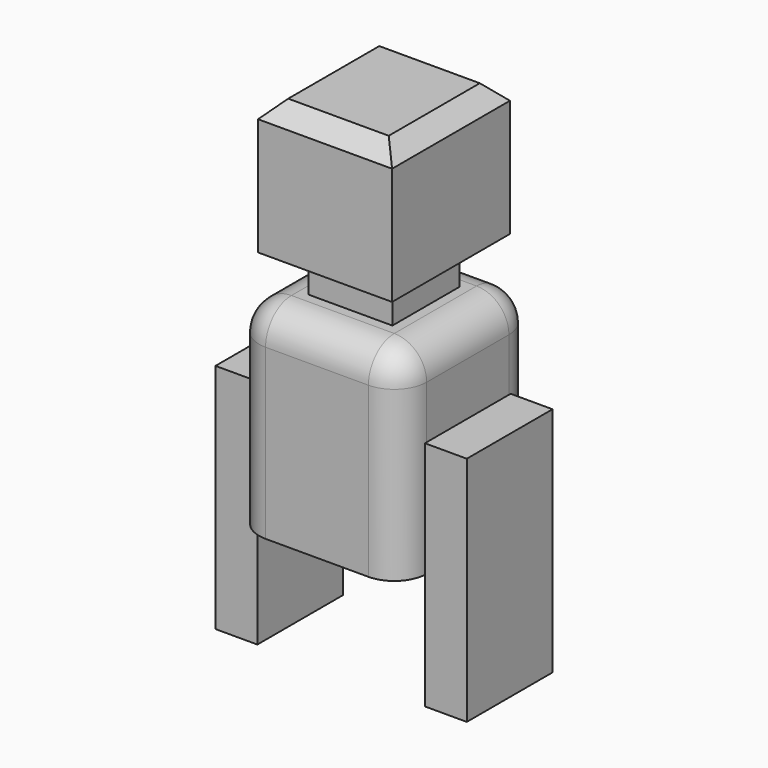
from build123d import *

# Parameters (mm, degrees)
F0_W      = 100
F0_H      = 100
F1_DEPTH  = 120
F2_W      = 50
F2_H      = 50
F3_DEPTH  = 50
F5_W      = 80
F5_H      = 87.9338901418
F6_DEPTH  = 80
F9_DEPTH  = 10
F10_W     = 63.9507248998
F10_H     = 69.1487565637
F11_DEPTH = 25
F14_R     = 19.313708499
F15_SIZE  = 10
F16_R     = 10
F17_DEPTH = 5
F20_R     = 5
F20_2_R   = 5


with BuildPart() as f1:
    # F0 (on Top) → F1 (new body)
    with BuildSketch(Plane.XY):
        Rectangle(F0_W, F0_H)
    extrude(amount=F1_DEPTH)

    # F2 (on face) → F3 (join)
    with BuildSketch(Plane.XY.offset(120)):
        Rectangle(F2_W, F2_H)
    extrude(amount=F3_DEPTH)


with BuildPart() as f6:
    # F5 (on offset) → F6 (new body)
    with BuildSketch(Plane.XY.offset(145)):
        Rectangle(F5_W, F5_H)
    extrude(amount=F6_DEPTH)

    # F7: cut F1
    add(f1.part, mode=Mode.SUBTRACT)

    # F15
    f15_edges = [f6.edges().sort_by_distance(p)[0] for p in [
        (-40, 0, 225),
        (0, 43.966945, 225),
        (40, 0, 225),
        (0, -43.966945, 225),
    ]]
    chamfer(f15_edges, length=F15_SIZE)


with BuildPart() as f9:
    # F8 (on face) → F9 (new body)
    with BuildSketch(Plane.YZ.offset(50)):
        with BuildLine():
            ThreePointArc((10, 40), (-7.0710678119, 47.0710678119), (0, 30))
            ThreePointArc((0, 30), (7.0710678119, 32.9289321881), (10, 40))
        make_face()
    extrude(amount=-F9_DEPTH)

    # F10 (on face) → F11 (join)
    with BuildSketch(Plane.YZ.offset(50)):
        with Locations((0, -34.5743782818)):
            Rectangle(F10_W, F10_H)
        with Locations((0, 34.5743782818)):
            Rectangle(F10_W, F10_H)
    extrude(amount=F11_DEPTH)


with BuildPart() as f1_1:
    add(f1.part)

    # F12: cut F9
    add(f9.part, mode=Mode.SUBTRACT)

    # F14
    f14_edges = [f1_1.edges().sort_by_distance(p)[0] for p in [
        (0, -50, 120),
        (-50, -50, 60),
        (50, -50, 60),
        (50, 50, 60),
        (0, 50, 120),
        (50, 0, 120),
        (-50, 50, 60),
        (-50, 0, 120),
    ]]
    fillet(f14_edges, radius=F14_R)


with BuildPart() as f13_1:
    # F13: instance of F9
    add(f9.part.mirror(Plane.YZ))


with BuildPart() as f17:
    # F16 (on face) → F17 (new body, symmetric)
    with BuildSketch(Plane(origin=(0, 43.9669450709, 0), x_dir=(-1, 0, 0), z_dir=(0, 1, 0))):
        with Locations((-19.5394717157, 182.368427515)):
            Circle(F16_R)
    extrude(amount=F17_DEPTH, both=True)


with BuildPart() as f18_1:
    # F18: instance of F17
    add(f17.part.mirror(Plane.YZ))


with BuildPart() as f6_1:
    add(f6.part)

    # F19: cut F17, F18_1
    add(f17.part, mode=Mode.SUBTRACT)
    add(f18_1.part, mode=Mode.SUBTRACT)


with BuildPart() as f17_1:
    add(f17.part)

    # F20
    f20_edges = [f17_1.edges().sort_by_distance(p)[0] for p in [
        (29.539472, 48.966945, 182.368428),
    ]]
    fillet(f20_edges, radius=F20_R)


with BuildPart() as f18_1_1:
    add(f18_1.part)

    # F20#2
    f20_2_edges = [f18_1_1.edges().sort_by_distance(p)[0] for p in [
        (-29.539472, 48.966945, 182.368428),
    ]]
    fillet(f20_2_edges, radius=F20_2_R)


solid = Compound([f9.part, f1_1.part, f13_1.part, f6_1.part, f17_1.part, f18_1_1.part])
